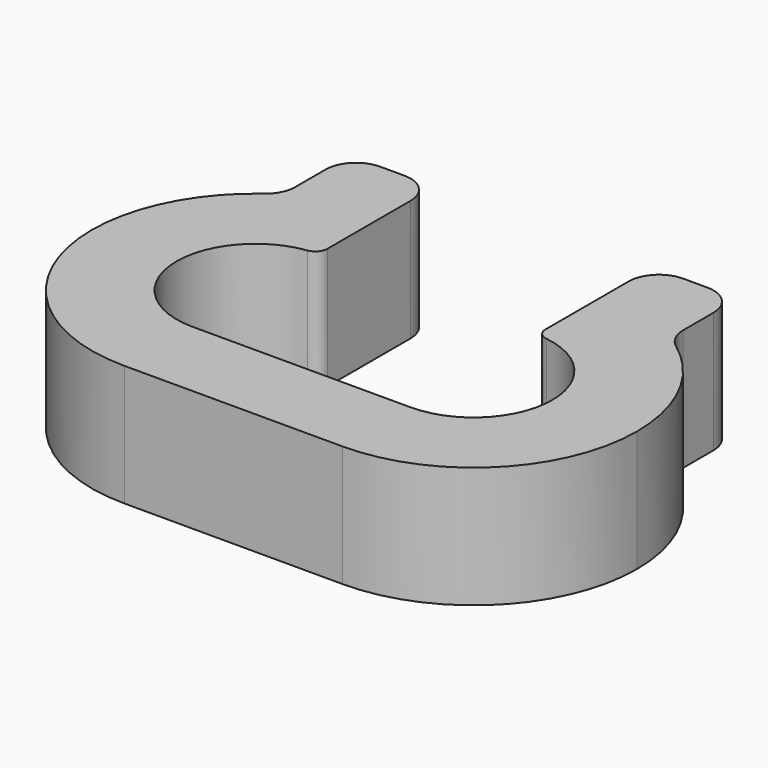
from build123d import *

# Parameters (mm, degrees)
F1_DEPTH = 10
F2_R     = 2.5
F3_R     = 1


with BuildPart() as f1:
    # F0 (on Top) → F1 (new body)
    with BuildSketch(Plane.XY):
        with BuildLine():
            ThreePointArc((15.5, 0), (13.5961940777, -4.5961940777), (9, -6.5))
            Line((9, -6.5), (2.8321595662, -6.5))
            ThreePointArc((2.8321595662, -6.5), (1.5672713544, -8.4013556122), (0, -10.0623058987))
            ThreePointArc((0, -10.0623058987), (4.1829017881, -12.611326846), (9, -13.5))
            ThreePointArc((9, -13.5), (18.545941546, -9.545941546), (22.5, 0))
            ThreePointArc((22.5, 0), (20.763290356, 6.6238206497), (16, 11.5433963806))
            ThreePointArc((16, 11.5433963806), (12.634153881, 13.0016508786), (9, 13.5))
            Line((9, 13.5), (9, 6.5))
            ThreePointArc((9, 6.5), (13.5961940777, 4.5961940777), (15.5, 0))
        make_face()
        with BuildLine():
            ThreePointArc((0, -10.0623058987), (1.5672713544, -8.4013556122), (2.8321595662, -6.5))
            Line((2.8321595662, -6.5), (-2.8321595662, -6.5))
            ThreePointArc((-2.8321595662, -6.5), (-1.5672713544, -8.4013556122), (0, -10.0623058987))
        make_face()
        with BuildLine():
            Line((9, 18.5), (9, 13.5))
            ThreePointArc((9, 13.5), (12.634153881, 13.0016508786), (16, 11.5433963806))
            Line((16, 11.5433963806), (16, 18.5))
            Line((16, 18.5), (9, 18.5))
        make_face()
        with BuildLine():
            ThreePointArc((0, -10.0623058987), (-1.5672713544, -8.4013556122), (-2.8321595662, -6.5))
            Line((-2.8321595662, -6.5), (-9, -6.5))
            ThreePointArc((-9, -6.5), (-15.5, 0), (-9, 6.5))
            Line((-9, 6.5), (-9, 13.5))
            ThreePointArc((-9, 13.5), (-12.634153881, 13.0016508786), (-16, 11.5433963806))
            ThreePointArc((-16, 11.5433963806), (-22.0016508786, -3.634153881), (-9, -13.5))
            ThreePointArc((-9, -13.5), (-4.1829017881, -12.611326846), (0, -10.0623058987))
        make_face()
        with BuildLine():
            ThreePointArc((9, -13.5), (4.1829017881, -12.611326846), (0, -10.0623058987))
            ThreePointArc((0, -10.0623058987), (-4.1829017881, -12.611326846), (-9, -13.5))
            Line((-9, -13.5), (9, -13.5))
        make_face()
        with BuildLine():
            ThreePointArc((-16, 11.5433963806), (-12.634153881, 13.0016508786), (-9, 13.5))
            Line((-9, 13.5), (-9, 18.5))
            Line((-9, 18.5), (-16, 18.5))
            Line((-16, 18.5), (-16, 11.5433963806))
        make_face()
    extrude(amount=F1_DEPTH)

    # F2
    f2_edges = [f1.edges().sort_by_distance(p)[0] for p in [
        (16, 18.5, 5),
        (9, 18.5, 5),
        (-9, 18.5, 5),
        (-16, 18.5, 5),
        (16, 11.543396, 5),
        (-16, 11.543396, 5),
    ]]
    fillet(f2_edges, radius=F2_R)

    # F3
    f3_edges = [f1.edges().sort_by_distance(p)[0] for p in [
        (-9, -6.5, 5),
        (9, -6.5, 5),
        (-9, 6.5, 5),
        (9, 6.5, 5),
    ]]
    fillet(f3_edges, radius=F3_R)


solid = f1.part
